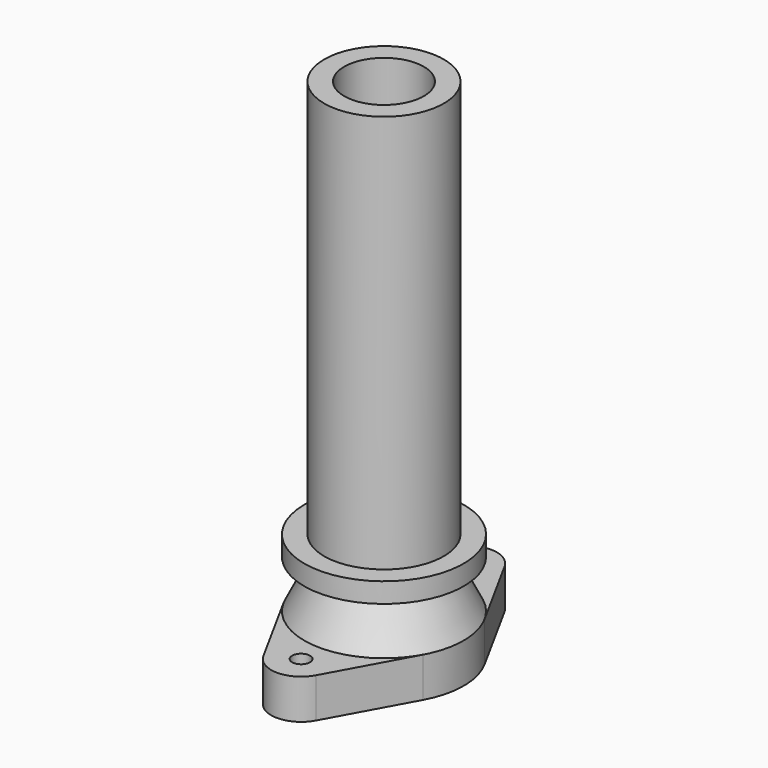
from build123d import *

# Parameters (mm, degrees)
F3_DEPTH  = 10
F0_W      = 2.95
F0_H      = 5
F0_W_2    = 2.9
F0_H_2    = 6
F7_DEPTH  = 10
F9_D      = 4.5
F10_SIZE2 = 9.99999
F10_SIZE  = 4.99999


# Not quite as in the source:
# - a fillet or chamfer is up to 0.001 mm smaller than in the source, because OpenCascade refuses the exact size
# - a feature of the source that left no trace in its solid (it failed there, or was rolled back) is left out


with BuildPart() as f1:
    # F0 (on Front) → F1 (revolve)
    with BuildSketch(Plane.XZ):
        Polygon((-20, 5), (-20, 0), (-6, 0), (-3.05, 0), (-3.05, 46), (-10, 46), (-10, 105), (-15, 105), (-15, 5), align=None)
    revolve(axis=Axis((0, 0, -11.1144582044), (0, 0, -1)))

    # F2 (on face) → F3 (cut)
    with BuildSketch(Plane.XY.offset(46)):
        Polygon((0, -6.0621778265), (5.25, -3.0310889132), (5.25, 3.0310889132), (0, 6.0621778265), (-5.25, 3.0310889132), (-5.25, -3.0310889132), align=None)
    extrude(amount=-F3_DEPTH, mode=Mode.SUBTRACT)


with BuildPart() as f4:
    # F0 (on Front) → F4 (revolve)
    with BuildSketch(Plane.XZ):
        with Locations((-4.525, -2.5)):
            Rectangle(F0_W, F0_H)
    revolve(axis=Axis((0, 0, -11.1144582044), (0, 0, -1)))


with BuildPart() as f5:
    # F0 (on Front) → F5 (revolve)
    with BuildSketch(Plane.XZ):
        Polygon((-9.65, -5), (-8, -2), (-20, -2), (-20, -22), (-9.65, -22), align=None)
    revolve(axis=Axis((0, 0, -11.1144582044), (0, 0, -1)))

    # F6 (on face) → F7 (join)
    with BuildSketch(Plane(origin=(0, 0, -22), x_dir=(1, 0, 0), z_dir=(0, 0, -1))):
        with BuildLine():
            ThreePointArc((-3.9275020998, -19.6105769231), (-11.8387740457, -16.1196597078), (-17.5369432541, -9.6153846154))
            Line((-17.5369432541, -9.6153846154), (-6.5763537203, -29.6057692308))
            ThreePointArc((-6.5763537203, -29.6057692308), (-7.249738898, -24.0787280488), (-3.9275020998, -19.6105769231))
        make_face()
        with BuildLine():
            ThreePointArc((-3.9275020998, -19.6105769231), (-7.249738898, -24.0787280488), (-6.5763537203, -29.6057692308))
            ThreePointArc((-6.5763537203, -29.6057692308), (0, -33.5), (6.5763537203, -29.6057692308))
            ThreePointArc((6.5763537203, -29.6057692308), (7.2654199088, -27.8610947179), (7.5, -26))
            ThreePointArc((7.5, -26), (6.5462304324, -22.3398268995), (3.9275020998, -19.6105769231))
            ThreePointArc((3.9275020998, -19.6105769231), (0, -20), (-3.9275020998, -19.6105769231))
        make_face()
        with BuildLine():
            Line((6.5763537203, -29.6057692308), (17.5369432541, -9.6153846154))
            ThreePointArc((17.5369432541, -9.6153846154), (11.8387740457, -16.1196597078), (3.9275020998, -19.6105769231))
            ThreePointArc((3.9275020998, -19.6105769231), (6.5462304324, -22.3398268995), (7.5, -26))
            ThreePointArc((7.5, -26), (7.2654199088, -27.8610947179), (6.5763537203, -29.6057692308))
        make_face()
        with BuildLine():
            ThreePointArc((3.9275020998, 19.6105769231), (6.5462304324, 22.3398268995), (7.5, 26))
            ThreePointArc((7.5, 26), (7.2654199088, 27.8610947179), (6.5763537203, 29.6057692308))
            ThreePointArc((6.5763537203, 29.6057692308), (0, 33.5), (-6.5763537203, 29.6057692308))
            ThreePointArc((-6.5763537203, 29.6057692308), (-7.249738898, 24.0787280488), (-3.9275020998, 19.6105769231))
            ThreePointArc((-3.9275020998, 19.6105769231), (0, 20), (3.9275020998, 19.6105769231))
        make_face()
        with BuildLine():
            ThreePointArc((6.5763537203, 29.6057692308), (7.2654199088, 27.8610947179), (7.5, 26))
            ThreePointArc((7.5, 26), (6.5462304324, 22.3398268995), (3.9275020998, 19.6105769231))
            ThreePointArc((3.9275020998, 19.6105769231), (11.8387740457, 16.1196597078), (17.5369432541, 9.6153846154))
            Line((17.5369432541, 9.6153846154), (6.5763537203, 29.6057692308))
        make_face()
        with BuildLine():
            ThreePointArc((-3.9275020998, 19.6105769231), (-7.249738898, 24.0787280488), (-6.5763537203, 29.6057692308))
            Line((-6.5763537203, 29.6057692308), (-17.5369432541, 9.6153846154))
            ThreePointArc((-17.5369432541, 9.6153846154), (-11.8387740457, 16.1196597078), (-3.9275020998, 19.6105769231))
        make_face()
    extrude(amount=-F7_DEPTH)

    # F9 (through all)
    with Locations(Plane.XY.offset(-12)):
        with Locations((0, -26), (0, 25)):
            Hole(F9_D / 2)

    # F10 (size 5 and 10 in the source; OpenCascade refuses exactly that, so slightly less here)
    f10_edges = [f5.edges().sort_by_distance(p)[0] for p in [
        (20, 0, -2),
    ]]
    chamfer(f10_edges, length=F10_SIZE, length2=F10_SIZE2)


with BuildPart() as f5b:
    # F0 (on Front) → F5, piece 2 (revolve)
    with BuildSketch(Plane.XZ):
        with Locations((-7.95, -19)):
            Rectangle(F0_W_2, F0_H_2)
    revolve(axis=Axis((0, 0, -11.1144582044), (0, 0, -1)))


solid = Compound([f1.part, f4.part, f5.part, f5b.part])
